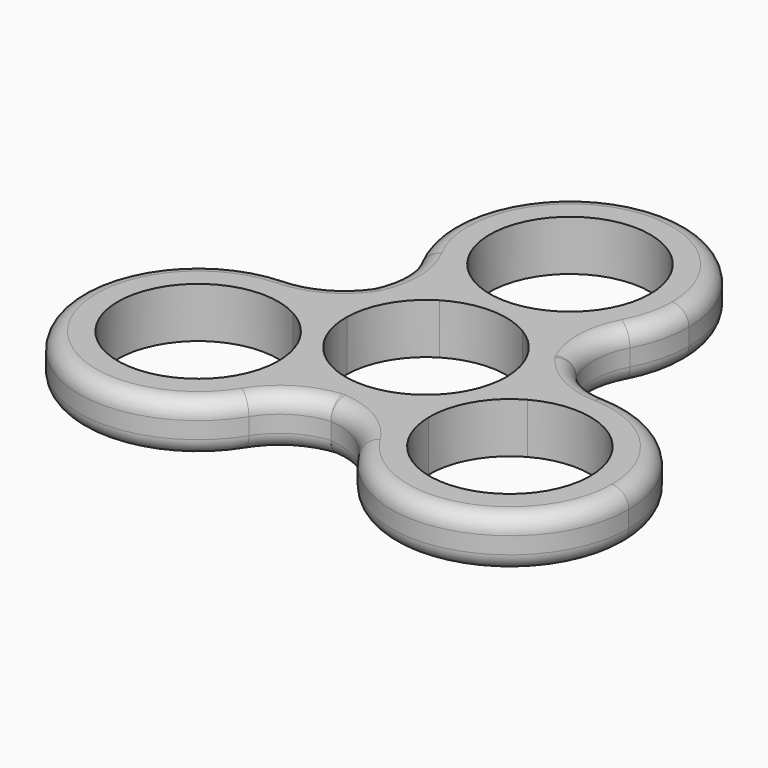
from build123d import *

# Parameters (mm, degrees)
F1_DEPTH    = 7
F2_T1_DEPTH = 7
F3_R        = 2.333


# Not quite as in the source:
# - a fillet or chamfer that OpenCascade refuses, or shapes differently, is made with other operations: its cross-section is extruded or revolved along the edge and cut away or added


with BuildPart() as f1:
    # F0 (on Top) → F1 (new body)
    with BuildSketch(Plane.XY):
        with BuildLine():
            ThreePointArc((11.1477191633, 0.2255159793), (11.1494297762, 0.1127637565), (11.15, 0))
            ThreePointArc((11.15, 0), (9.5993075457, -5.6723711659), (5.3785570146, -9.7669659793))
            ThreePointArc((5.3785570146, -9.7669659793), (5.1515621474, -12.6749053564), (5.4401527402, -15.5773790531))
            ThreePointArc((5.4401527402, -15.5773790531), (8.0980639917, -14.3760689893), (10.5029159313, -12.7255159793))
            ThreePointArc((10.5029159313, -12.7255159793), (11.9944518424, -6.925), (16.27207808, -2.7330340207))
            ThreePointArc((16.27207808, -2.7330340207), (16.4429207916, -1.3712606754), (16.5, 0))
            ThreePointArc((16.5, 0), (16.4274611375, 1.5454839293), (16.2104823544, 3.0773790531))
            ThreePointArc((16.2104823544, 3.0773790531), (13.5525711029, 1.8760689893), (11.1477191633, 0.2255159793))
        make_face()
        with BuildLine():
            ThreePointArc((5.7691621487, 9.54145), (9.6561832522, 5.575), (11.1477191633, 0.2255159793))
            ThreePointArc((11.1477191633, 0.2255159793), (13.5525711029, 1.8760689893), (16.2104823544, 3.0773790531))
            ThreePointArc((16.2104823544, 3.0773790531), (14.2894191624, 8.25), (10.7703296143, 12.5))
            ThreePointArc((10.7703296143, 12.5), (8.4010089555, 10.798836367), (5.7691621487, 9.54145))
        make_face()
        with BuildLine():
            ThreePointArc((5.4401527402, -15.5773790531), (5.1515621474, -12.6749053564), (5.3785570146, -9.7669659793))
            ThreePointArc((5.3785570146, -9.7669659793), (0, -11.15), (-5.3785570146, -9.7669659793))
            ThreePointArc((-5.3785570146, -9.7669659793), (-5.207714303, -11.1287393246), (-5.1506350946, -12.5))
            ThreePointArc((-5.1506350946, -12.5), (-5.2231739571, -14.0454839293), (-5.4401527402, -15.5773790531))
            ThreePointArc((-5.4401527402, -15.5773790531), (0, -16.5), (5.4401527402, -15.5773790531))
        make_face()
        with BuildLine():
            ThreePointArc((-5.7691621487, 9.54145), (0, 11.15), (5.7691621487, 9.54145))
            ThreePointArc((5.7691621487, 9.54145), (8.4010089555, 10.798836367), (10.7703296143, 12.5))
            ThreePointArc((10.7703296143, 12.5), (8.4010089555, 14.201163633), (5.7691621487, 15.45855))
            ThreePointArc((5.7691621487, 15.45855), (0, 13.85), (-5.7691621487, 15.45855))
            ThreePointArc((-5.7691621487, 15.45855), (-8.4010089555, 14.201163633), (-10.7703296143, 12.5))
            ThreePointArc((-10.7703296143, 12.5), (-8.4010089555, 10.798836367), (-5.7691621487, 9.54145))
        make_face()
        with BuildLine():
            ThreePointArc((38.1506350946, -12.5), (31.2027940073, 0.9538567001), (16.2104823544, 3.0773790531))
            ThreePointArc((16.2104823544, 3.0773790531), (16.4274611375, 1.5454839293), (16.5, 0))
            ThreePointArc((16.5, 0), (16.4429207916, -1.3712606754), (16.27207808, -2.7330340207))
            ThreePointArc((16.27207808, -2.7330340207), (27.3230062605, -2.9006924543), (32.8006350946, -12.5))
            ThreePointArc((32.8006350946, -12.5), (21.7633988511, -23.6494297762), (10.5029159313, -12.7255159793))
            ThreePointArc((10.5029159313, -12.7255159793), (8.0980639917, -14.3760689893), (5.4401527402, -15.5773790531))
            ThreePointArc((5.4401527402, -15.5773790531), (23.196119024, -28.9274611375), (38.1506350946, -12.5))
        make_face()
        with BuildLine():
            ThreePointArc((-5.1506350946, -12.5), (-5.207714303, -11.1287393246), (-5.3785570146, -9.7669659793))
            ThreePointArc((-5.3785570146, -9.7669659793), (-7.8041013842, -7.963573418), (-9.6561832522, -5.575))
            Line((-9.6561832522, -5.575), (-11.9944518424, -6.925))
            ThreePointArc((-11.9944518424, -6.925), (-10.8805621315, -9.6141676471), (-10.5006350946, -12.5))
            ThreePointArc((-10.5006350946, -12.5), (-10.5012053184, -12.6127637565), (-10.5029159313, -12.7255159793))
            ThreePointArc((-10.5029159313, -12.7255159793), (-8.0980639917, -14.3760689893), (-5.4401527402, -15.5773790531))
            ThreePointArc((-5.4401527402, -15.5773790531), (-5.2231739571, -14.0454839293), (-5.1506350946, -12.5))
        make_face()
        with BuildLine():
            ThreePointArc((-11.1477191633, 0.2255159793), (-9.6561832522, 5.575), (-5.7691621487, 9.54145))
            ThreePointArc((-5.7691621487, 9.54145), (-8.4010089555, 10.798836367), (-10.7703296143, 12.5))
            ThreePointArc((-10.7703296143, 12.5), (-14.2894191624, 8.25), (-16.2104823544, 3.0773790531))
            ThreePointArc((-16.2104823544, 3.0773790531), (-13.5525711029, 1.8760689893), (-11.1477191633, 0.2255159793))
        make_face()
        with BuildLine():
            ThreePointArc((5.7691621487, 15.45855), (8.4010089555, 14.201163633), (10.7703296143, 12.5))
            ThreePointArc((10.7703296143, 12.5), (14.9993406294, 18.1246977752), (16.5, 25))
            ThreePointArc((16.5, 25), (-6.8753022248, 39.9993406294), (-10.7703296143, 12.5))
            ThreePointArc((-10.7703296143, 12.5), (-8.4010089555, 14.201163633), (-5.7691621487, 15.45855))
            ThreePointArc((-5.7691621487, 15.45855), (-5.4770586104, 34.7120713022), (11.15, 25))
            ThreePointArc((11.15, 25), (9.7120713022, 19.5229413896), (5.7691621487, 15.45855))
        make_face()
        with BuildLine():
            Line((-11.9944518424, -6.925), (-9.6561832522, -5.575))
            ThreePointArc((-9.6561832522, -5.575), (-10.798707577, -2.7767633434), (-11.1477191633, 0.2255159793))
            ThreePointArc((-11.1477191633, 0.2255159793), (-13.5525711029, 1.8760689893), (-16.2104823544, 3.0773790531))
            ThreePointArc((-16.2104823544, 3.0773790531), (-16.4990729472, 0.1749053564), (-16.27207808, -2.7330340207))
            ThreePointArc((-16.27207808, -2.7330340207), (-13.8465337104, -4.536426582), (-11.9944518424, -6.925))
        make_face()
        with BuildLine():
            ThreePointArc((-16.2104823544, 3.0773790531), (-35.9400542571, -20.75), (-5.4401527402, -15.5773790531))
            ThreePointArc((-5.4401527402, -15.5773790531), (-8.0980639917, -14.3760689893), (-10.5029159313, -12.7255159793))
            ThreePointArc((-10.5029159313, -12.7255159793), (-31.3068183468, -18.075), (-16.27207808, -2.7330340207))
            ThreePointArc((-16.27207808, -2.7330340207), (-16.4990729472, 0.1749053564), (-16.2104823544, 3.0773790531))
        make_face()
    extrude(amount=F1_DEPTH)

    # F2: fillet of radius 10 on 6 edges, made by hand

    # F2_s2 → F2_t1 (join)
    with BuildSketch(Plane.XY):
        with BuildLine():
            ThreePointArc((-7.6358221368, -21.2083303657), (-4.1419961018, -17.825852307), (0.5342288423, -16.4913492336))
            ThreePointArc((0.5342288423, -16.4913492336), (-2.4951668673, -16.3102465433), (-5.4401527402, -15.5773790531))
            ThreePointArc((-5.4401527402, -15.5773790531), (-6.2779638124, -18.4942453779), (-7.6358221368, -21.2083303657))
        make_face()
        with BuildLine():
            ThreePointArc((-14.5490418001, 17.2169811321), (-13.3666428911, 12.5), (-14.5490418001, 7.7830188679))
            ThreePointArc((-14.5490418001, 7.7830188679), (-12.8775044149, 10.3160011654), (-10.7703296143, 12.5))
            ThreePointArc((-10.7703296143, 12.5), (-12.8775044149, 14.6839988346), (-14.5490418001, 17.2169811321))
        make_face()
        with BuildLine():
            ThreePointArc((14.5490418001, 7.7830188679), (13.3666428911, 12.5), (14.5490418001, 17.2169811321))
            ThreePointArc((14.5490418001, 17.2169811321), (12.8775044149, 14.6839988346), (10.7703296143, 12.5))
            ThreePointArc((10.7703296143, 12.5), (12.8775044149, 10.3160011654), (14.5490418001, 7.7830188679))
        make_face()
        with BuildLine():
            ThreePointArc((-0.5342288423, -16.4913492336), (4.1419961018, -17.825852307), (7.6358221368, -21.2083303657))
            ThreePointArc((7.6358221368, -21.2083303657), (6.2779638124, -18.4942453779), (5.4401527402, -15.5773790531))
            ThreePointArc((5.4401527402, -15.5773790531), (2.4951668673, -16.3102465433), (-0.5342288423, -16.4913492336))
        make_face()
        with BuildLine():
            ThreePointArc((14.0148129578, 8.7083303657), (17.5086389929, 5.325852307), (22.1848639369, 3.9913492336))
            ThreePointArc((22.1848639369, 3.9913492336), (19.1554682273, 3.8102465433), (16.2104823544, 3.0773790531))
            ThreePointArc((16.2104823544, 3.0773790531), (15.3726712822, 5.9942453779), (14.0148129578, 8.7083303657))
        make_face()
        with BuildLine():
            ThreePointArc((-14.0148129578, 8.7083303657), (-17.5086389929, 5.325852307), (-22.1848639369, 3.9913492336))
            ThreePointArc((-22.1848639369, 3.9913492336), (-19.1554682273, 3.8102465433), (-16.2104823544, 3.0773790531))
            ThreePointArc((-16.2104823544, 3.0773790531), (-15.3726712822, 5.9942453779), (-14.0148129578, 8.7083303657))
        make_face()
    extrude(amount=F2_T1_DEPTH)

    # F3 (call 1 of 2: OpenCascade refuses the feature's edges together)
    f3_edges = [f1.edges().sort_by_distance(p)[0] for p in [
        (0, 41.5, 7),
        (-13.370224, 12.767582, 7),
        (-4.371939, -17.962744, 7),
        (-35.940054, -20.75, 7),
        (17.742162, 5.195162, 7),
        (35.940054, -20.75, 7),
        (-17.742162, 5.195162, 7),
        (4.371939, -17.962744, 7),
        (13.370224, 12.767582, 7),
    ]]
    fillet(f3_edges, radius=F3_R)

    # F3#2 (call 2 of 2)
    f3_2_edges = [f1.edges().sort_by_distance(p)[0] for p in [
        (-35.940054, -20.75, 0),
        (-17.742162, 5.195162, 0),
        (35.940054, -20.75, 0),
        (4.371939, -17.962744, 0),
        (13.370224, 12.767582, 0),
        (0, 41.5, 0),
        (-13.370224, 12.767582, 0),
        (-4.371939, -17.962744, 0),
        (17.742162, 5.195162, 0),
    ]]
    fillet(f3_2_edges, radius=F3_R)


solid = f1.part
